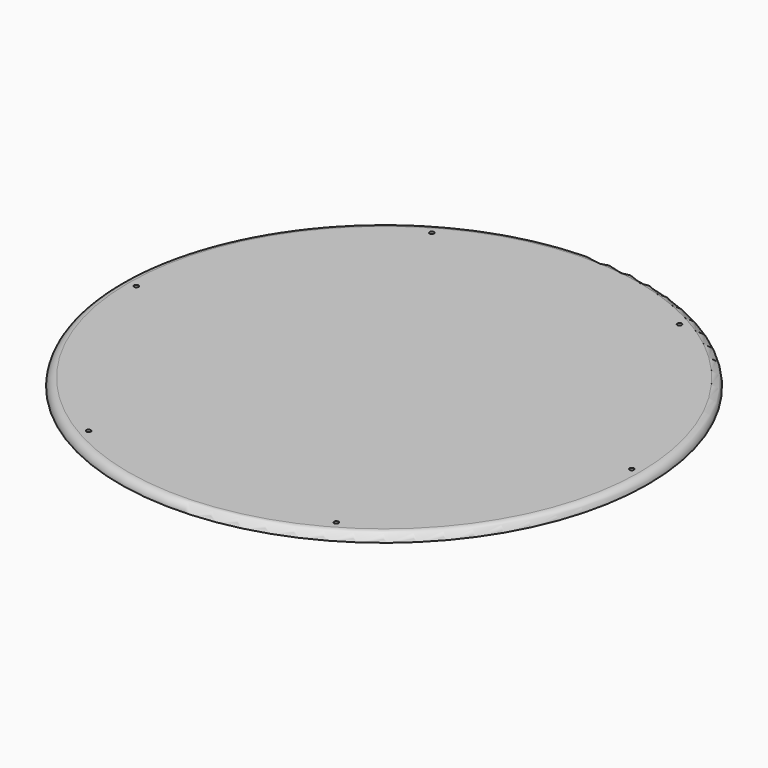
from build123d import *

# Parameters (mm, degrees)
F0_R     = 206.5196172612
F0_R_2   = 1.7272
F1_DEPTH = 6.35
F2_R     = 6.34999


# Not quite as in the source:
# - a fillet or chamfer is up to 0.001 mm smaller than in the source, because OpenCascade refuses the exact size


with BuildPart() as f1:
    # F0 (on Top) → F1 (new body)
    with BuildSketch(Plane.XY):
        Circle(F0_R)
        with Locations((-96.9098086306, -167.8527123)):
            Circle(F0_R_2, mode=Mode.SUBTRACT)
        with Locations((96.9098086306, -167.8527123)):
            Circle(F0_R_2, mode=Mode.SUBTRACT)
        with Locations((-193.8196172612, 0)):
            Circle(F0_R_2, mode=Mode.SUBTRACT)
        with Locations((-96.9098086306, 167.8527123)):
            Circle(F0_R_2, mode=Mode.SUBTRACT)
        with Locations((193.8196172612, 0)):
            Circle(F0_R_2, mode=Mode.SUBTRACT)
        with Locations((96.9098086306, 167.8527123)):
            Circle(F0_R_2, mode=Mode.SUBTRACT)
    extrude(amount=F1_DEPTH)

    # F2 (radius 6.35 in the source; OpenCascade refuses exactly that, so slightly less here)
    f2_edges = [f1.edges().sort_by_distance(p)[0] for p in [
        (-206.519617, 0, 6.35),
    ]]
    fillet(f2_edges, radius=F2_R)


solid = f1.part
